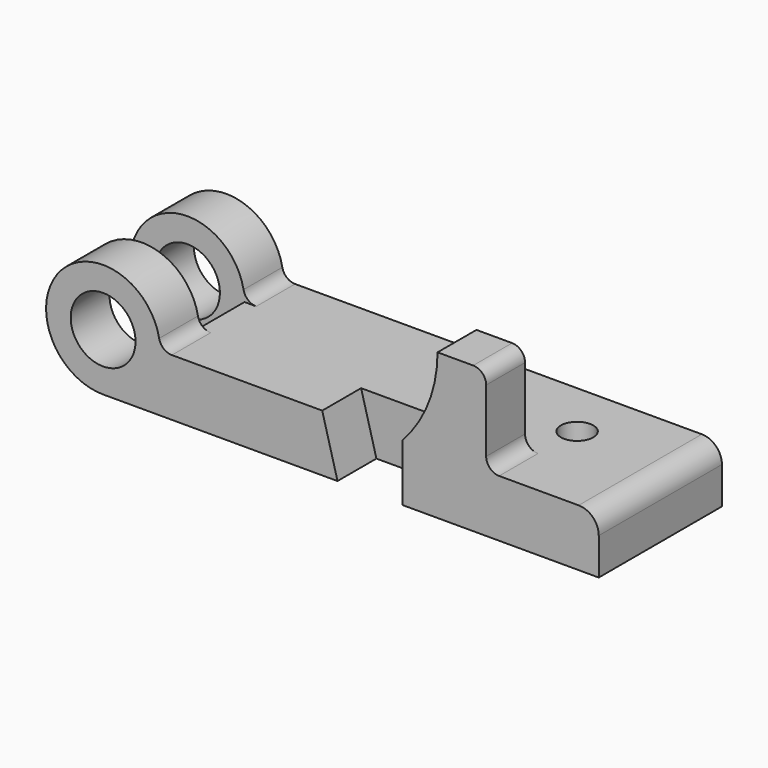
from build123d import *

# Parameters (mm, degrees)
F0_R          = 12.7
F0_W          = 76.962
F0_H          = 22.352
F1_DEPTH      = 30.1625
F2_W          = 44.704
F2_H          = 22.3266
F3_DEPTH      = 22.353
F3_DEPTH_BACK = 22.353
F2_R          = 6.35
F4_DEPTH      = 22.353
F6_DEPTH      = 19.05
F8_DEPTH      = 19.05
F9_R          = 7.874
F10_R         = 5.08


with BuildPart() as f1:
    # F0 (on Front) → F1 (new body, symmetric)
    with BuildSketch(Plane.XZ):
        with BuildLine():
            ThreePointArc((0, -22.352), (15.8052507731, -15.8052507731), (22.352, 0))
            ThreePointArc((22.352, 0), (-15.8052507731, 15.8052507731), (0, -22.352))
        make_face()
        Circle(F0_R, mode=Mode.SUBTRACT)
        with BuildLine():
            Line((85.852, 0), (22.352, 0))
            ThreePointArc((22.352, 0), (15.8052507731, -15.8052507731), (0, -22.352))
            Line((0, -22.352), (91.8464, -22.352))
            Line((91.8464, -22.352), (85.852, 0))
        make_face()
        with Locations((155.7274, -11.176)):
            Rectangle(F0_W, F0_H)
        Polygon((117.2464, 0), (85.852, 0), (91.8464, -22.352), (117.2464, -22.352), align=None)
    extrude(amount=F1_DEPTH, both=True)

    # F2 (on face) → F3 (cut, two sides)
    with BuildSketch(Plane.XY) as f3_sk:
        Rectangle(F2_W, F2_H)
    extrude(amount=F3_DEPTH, mode=Mode.SUBTRACT)
    extrude(f3_sk.sketch, amount=-F3_DEPTH_BACK, mode=Mode.SUBTRACT)

    # F2 (on face) → F4 (cut, through all)
    with BuildSketch(Plane.XY):
        with Locations((155.3464, 7.8105)):
            Circle(F2_R)
    extrude(amount=-F4_DEPTH, mode=Mode.SUBTRACT)

    # F5 (on face) → F6 (cut)
    with BuildSketch(Plane.XZ.offset(30.1625)):
        Polygon((117.2464, 0), (85.852, 0), (91.8464, -22.352), (117.2464, -22.352), align=None)
    extrude(amount=-F6_DEPTH, mode=Mode.SUBTRACT)

    # F7 (on face) → F8 (join)
    with BuildSketch(Plane.XZ.offset(30.1625)):
        with BuildLine():
            Line((117.2464, 0), (150.0886, 0))
            Line((150.0886, 0), (150.0886, 34.798))
            Line((150.0886, 34.798), (131.0386, 34.798))
            ThreePointArc((131.0386, 34.798), (127.4644153616, 16.0823576341), (117.2464, 0))
        make_face()
    extrude(amount=-F8_DEPTH)

    # F9
    f9_edges = [f1.edges().sort_by_distance(p)[0] for p in [
        (194.2084, 0, 0),
    ]]
    fillet(f9_edges, radius=F9_R)

    # F10
    f10_edges = [f1.edges().sort_by_distance(p)[0] for p in [
        (150.0886, -20.6375, 34.798),
        (150.0886, -20.6375, 0),
        (22.352, 20.6629, 0),
        (22.352, -20.6629, 0),
    ]]
    fillet(f10_edges, radius=F10_R)


solid = f1.part
